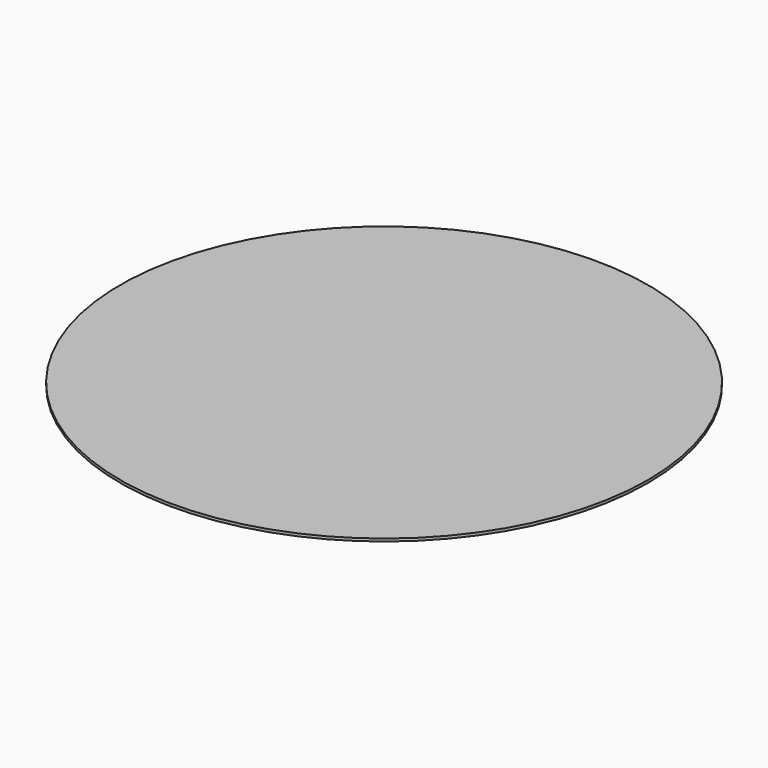
from build123d import *

# Parameters (mm, degrees)
F0_R     = 2495.0806395664
F2_DEPTH = 25


# Not quite as in the source:
# - the program builds the solid bodies; features that only make, move or delete a surface that nothing else refers to are left out


with BuildPart() as f2:
    # F0 (on Top) → F2 (new body)
    with BuildSketch(Plane.XY):
        Circle(F0_R)
    extrude(amount=F2_DEPTH)


solid = f2.part
